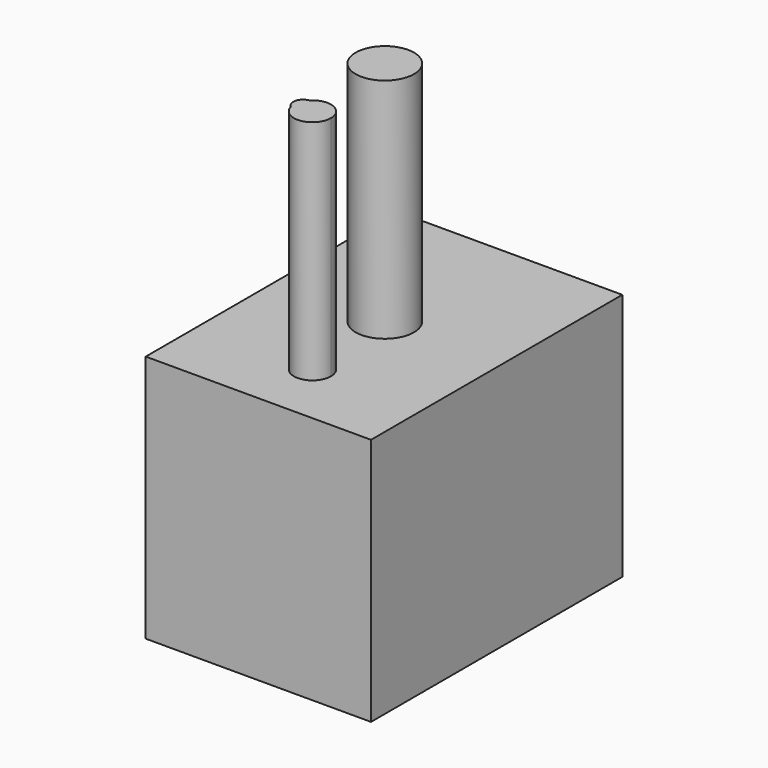
from build123d import *

# Parameters (mm, degrees)
F0_W     = 78.2610476017
F0_H     = 61.8856586516
F1_DEPTH = 56.134
F4_R     = 7.271205843
F5_DEPTH = 56.642


# Not quite as in the source:
# - the program builds the solid bodies; features that only make, move or delete a surface that nothing else refers to are left out


with BuildPart() as f1:
    # F0 (on Right) → F1 (new body)
    with BuildSketch(Plane.YZ):
        with Locations((39.1305238008, -30.9428293258)):
            Rectangle(F0_W, F0_H)
    extrude(amount=F1_DEPTH)

    # F4 (on face) → F5 (join)
    with BuildSketch(Plane.XY):
        with Locations((27.1040890366, 40.5922196805)):
            Circle(F4_R)
        with BuildLine():
            ThreePointArc((24.2466891936, 14.9025116275), (26.8248957449, 14.6298549046), (28.1992270717, 16.8281961232))
            ThreePointArc((28.1992270717, 16.8281961232), (27.3655770879, 18.6672690129), (25.4330261647, 19.2524256742))
            ThreePointArc((25.4330261647, 19.2524256742), (24.2724174076, 17.232224668), (24.2466891936, 14.9025116275))
        make_face()
        with BuildLine():
            ThreePointArc((25.4330261647, 19.2524256742), (27.3655770879, 18.6672690129), (28.1992270717, 16.8281961232))
            ThreePointArc((28.1992270717, 16.8281961232), (26.8248957449, 14.6298549046), (24.2466891936, 14.9025116275))
            ThreePointArc((24.2466891936, 14.9025116275), (29.2863202966, 11.4378625234), (33.3389067896, 16.0180609673))
            ThreePointArc((33.3389067896, 16.0180609673), (30.4716460582, 20.2890111986), (25.4330261647, 19.2524256742))
        make_face()
        with BuildLine():
            ThreePointArc((24.2466891936, 14.9025116275), (24.2724174076, 17.232224668), (25.4330261647, 19.2524256742))
            ThreePointArc((25.4330261647, 19.2524256742), (23.394656757, 17.4716132859), (24.2466891936, 14.9025116275))
        make_face()
    extrude(amount=F5_DEPTH)


solid = f1.part
